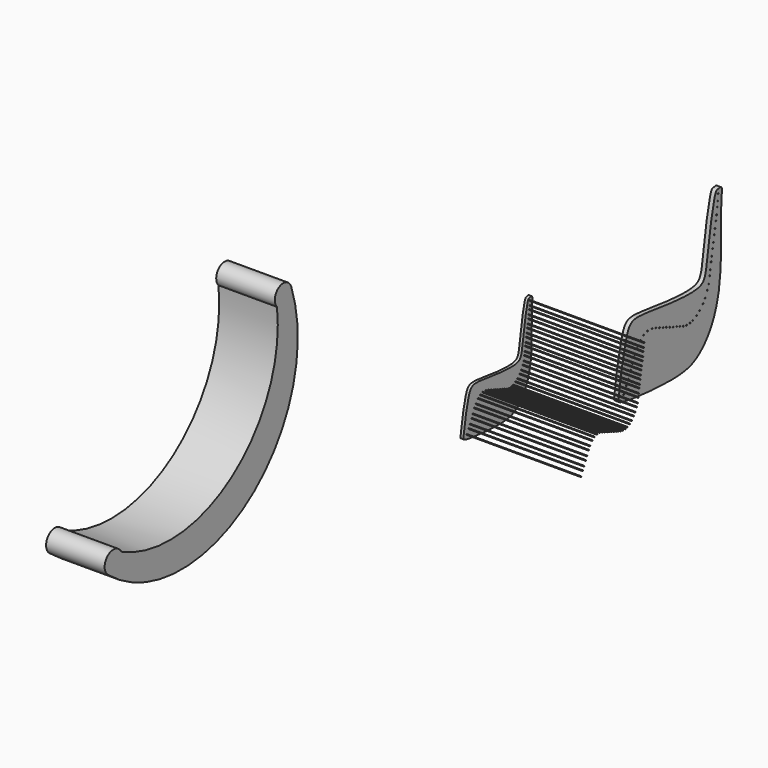
from build123d import *

# Parameters (mm, degrees)
F2_DEPTH = 127
F4_DEPTH = 12.7
F5_SCALE = 1.5
F6_DEPTH = 508


# Not quite as in the source:
# - a feature names something its author has since deleted; it is built from what else it names


with BuildPart() as f2:
    # F1 (on Right) → F2 (new body, symmetric)
    with BuildSketch(Plane.YZ):
        with BuildLine():
            ThreePointArc((-405.3666641437, -282.9348817468), (-431.1960064464, -325.2227693858), (-480.6119799614, -321.5509951115))
            ThreePointArc((-480.6119799614, -321.5509951115), (278.9839250065, -347.7055505892), (511.339366436, 375.9524822235))
            ThreePointArc((511.339366436, 375.9524822235), (513.173736402, 368.6540148527), (513.7907227287, 361.1538903865))
            ThreePointArc((513.7907227287, 361.1538903865), (484.5631181842, 318.392706642), (434.1071248055, 330.0958871841))
            ThreePointArc((434.1071248055, 330.0958871841), (189.1196757774, -218.9533749106), (-410.6203019619, -261.2133026123))
            ThreePointArc((-410.6203019619, -261.2133026123), (-406.6987393278, -271.7609420832), (-405.3666641437, -282.9348817468))
        make_face()
        with BuildLine():
            ThreePointArc((-410.6203019619, -261.2133026123), (-483.9335544164, -246.9339780219), (-480.6119799614, -321.5509951115))
            ThreePointArc((-480.6119799614, -321.5509951115), (-431.1960064464, -325.2227693858), (-405.3666641437, -282.9348817468))
            ThreePointArc((-405.3666641437, -282.9348817468), (-406.6987393278, -271.7609420832), (-410.6203019619, -261.2133026123))
        make_face()
        with BuildLine():
            ThreePointArc((513.7907227287, 361.1538903865), (513.173736402, 368.6540148527), (511.339366436, 375.9524822235))
            ThreePointArc((511.339366436, 375.9524822235), (444.4653431931, 400.6164916858), (434.1071248055, 330.0958871841))
            ThreePointArc((434.1071248055, 330.0958871841), (484.5631181842, 318.392706642), (513.7907227287, 361.1538903865))
        make_face()
    extrude(amount=F2_DEPTH, both=True)


with BuildPart() as f4:
    # F3 (on Right) → F4 (new body)
    with BuildSketch(Plane.YZ):
        with BuildLine():
            add(Edge.make_bspline(
                [(1588.1042480469, -672.3895072937), (1590.7751967656, -646.3995932049), (1611.7959010002, -517.5506212092), (1641.7401584726, -489.021724859), (1720.9312550677, -500.8093748422), (1881.0798668429, -519.9918232799), (1904.7947275082, -486.1107940737), (1911.014539794, -415.1749746357), (1934.8258228227, -286.8214563677), (1945.6474567466, -286.2346451362), (1965.0613414177, -281.763240351), (1954.2066132557, -330.1428987209), (1965.6410866407, -524.5072510181), (1926.7903882604, -626.0098057417), (1895.9895754535, -664.9340201656), (1851.033974807, -703.2355431509), (1742.9778221098, -706.2354101889), (1588.1977710336, -690.3922627167), (1587.3192204388, -680.0282912013), (1588.1042480469, -672.3895072937)],
                knots=[0, 0, 0, 0, 0.086766165, 0.1291659204, 0.191487798, 0.2795961904, 0.3179244262, 0.3798889709, 0.4579456316, 0.4772361122, 0.5017320687, 0.543105293, 0.6429735253, 0.7164751466, 0.7638864843, 0.8141635884, 0.8901962157, 0.9744982618, 1, 1, 1, 1], degree=3))
        make_face()
        with BuildLine():
            ThreePointArc((1607.8116078098, -670.6807075021), (1604.8770943632, -671.5207735855), (1606.9225230544, -669.2550945124))
            ThreePointArc((1606.9225230544, -669.2550945124), (1607.5711212565, -669.8406414186), (1607.8116078098, -670.6807075021))
        make_face(mode=Mode.SUBTRACT)
        with BuildLine():
            ThreePointArc((1617.2146263828, -651.7951774392), (1616.4601126896, -653.1465804371), (1614.9137885085, -653.2133824057))
            ThreePointArc((1614.9137885085, -653.2133824057), (1614.2090096098, -651.0816642522), (1616.3408148715, -650.3771488812))
            ThreePointArc((1616.3408148715, -650.3771488812), (1616.9786323439, -650.9623581988), (1617.2146263828, -651.7951774392))
        make_face(mode=Mode.SUBTRACT)
        with BuildLine():
            ThreePointArc((1624.441297583, -637.4331976519), (1623.6873478332, -638.7842528803), (1622.1416437494, -638.8519975557))
            ThreePointArc((1622.1416437494, -638.8519975557), (1621.4348029778, -636.7214318474), (1623.5651753051, -636.0140084515))
            ThreePointArc((1623.5651753051, -636.0140084515), (1624.2046248081, -636.5992779566), (1624.441297583, -637.4331976519))
        make_face(mode=Mode.SUBTRACT)
        with BuildLine():
            ThreePointArc((1633.4229065248, -619.2392863847), (1632.6790615082, -620.5840549591), (1631.1446041388, -620.6686038139))
            ThreePointArc((1631.1446041388, -620.6686038139), (1630.4054246212, -618.5498605326), (1632.5234552037, -617.8086413325))
            ThreePointArc((1632.5234552037, -617.8086413325), (1633.1793621654, -618.3943369861), (1633.4229065248, -619.2392863847))
        make_face(mode=Mode.SUBTRACT)
        with BuildLine():
            ThreePointArc((1640.1858726451, -604.7830555746), (1639.4584529937, -606.1173786404), (1637.9428262905, -606.2288824062))
            ThreePointArc((1637.9428262905, -606.2288824062), (1637.1518979459, -604.1289399927), (1639.251056814, -603.3359344236))
            ThreePointArc((1639.251056814, -603.3359344236), (1639.9318441237, -603.9216555131), (1640.1858726451, -604.7830555746))
        make_face(mode=Mode.SUBTRACT)
        with BuildLine():
            ThreePointArc((1648.8267409237, -585.9965814537), (1648.0802623737, -587.3429986144), (1646.5428490552, -587.4231839266))
            ThreePointArc((1646.5428490552, -587.4231839266), (1645.8151480681, -585.295071804), (1647.9458593109, -584.5750165748))
            ThreePointArc((1647.9458593109, -584.5750165748), (1648.5886691248, -585.1603997868), (1648.8267409237, -585.9965814537))
        make_face(mode=Mode.SUBTRACT)
        with BuildLine():
            ThreePointArc((1656.0821342109, -572.7840732335), (1655.2700718309, -574.1692998386), (1653.6646819307, -574.1373416705))
            ThreePointArc((1653.6646819307, -574.1373416705), (1653.147010351, -571.944986717), (1655.3428165759, -571.4421556035))
            ThreePointArc((1655.3428165759, -571.4421556035), (1655.8850740252, -572.0180227308), (1656.0821342109, -572.7840732335))
        make_face(mode=Mode.SUBTRACT)
        with BuildLine():
            ThreePointArc((1668.1439102008, -557.277738545), (1667.1696433417, -558.7420135755), (1665.4426801347, -558.4090040266))
            ThreePointArc((1665.4426801347, -558.4090040266), (1665.4394903681, -556.1496222667), (1667.6987279241, -556.1753472946))
            ThreePointArc((1667.6987279241, -556.1753472946), (1668.028413196, -556.6832947443), (1668.1439102008, -557.277738545))
        make_face(mode=Mode.SUBTRACT)
        with BuildLine():
            ThreePointArc((1680.1075762918, -548.3992204924), (1678.9093390409, -549.9382561522), (1677.1234745442, -549.1539786049))
            ThreePointArc((1677.1234745442, -549.1539786049), (1677.7903828704, -546.9893610097), (1679.9427437215, -547.6948245564))
            ThreePointArc((1679.9427437215, -547.6948245564), (1680.0658189603, -548.0375081029), (1680.1075762918, -548.3992204924))
        make_face(mode=Mode.SUBTRACT)
        with BuildLine():
            ThreePointArc((1694.1690954304, -543.8397874236), (1692.7157248498, -545.4216109121), (1691.0167608806, -544.1070870345))
            ThreePointArc((1691.0167608806, -544.1070870345), (1692.3410507485, -542.2706174181), (1694.1546434805, -543.6260677893))
            ThreePointArc((1694.1546434805, -543.6260677893), (1694.1654783221, -543.732683571), (1694.1690954304, -543.8397874236))
        make_face(mode=Mode.SUBTRACT)
        with BuildLine():
            ThreePointArc((1710.5441406901, -544.5462468817), (1708.6919971387, -545.7888023035), (1707.4253199722, -543.9530712046))
            ThreePointArc((1707.4253199722, -543.9530712046), (1709.127233525, -542.647822494), (1710.5761103558, -544.2292585082))
            ThreePointArc((1710.5761103558, -544.2292585082), (1710.5680977181, -544.3885567257), (1710.5441406901, -544.5462468817))
        make_face(mode=Mode.SUBTRACT)
        with BuildLine():
            ThreePointArc((1737.2629255193, -553.4428964877), (1735.2296018425, -554.3961653446), (1734.277468412, -552.3623097405))
            ThreePointArc((1734.277468412, -552.3623097405), (1736.0446029311, -551.3398854822), (1737.3573953003, -552.9034365583))
            ThreePointArc((1737.3573953003, -552.9034365583), (1737.3335995119, -553.1772711594), (1737.2629255193, -553.4428964877))
        make_face(mode=Mode.SUBTRACT)
        with BuildLine():
            ThreePointArc((1724.2944062995, -548.7008975511), (1722.2714523473, -549.6646490244), (1721.3000207205, -547.645371879))
            ThreePointArc((1721.3000207205, -547.645371879), (1723.0639632017, -546.6021765173), (1724.3867189937, -548.1674454253))
            ThreePointArc((1724.3867189937, -548.1674454253), (1724.3634705876, -548.438135656), (1724.2944062995, -548.7008975511))
        make_face(mode=Mode.SUBTRACT)
        with BuildLine():
            ThreePointArc((1774.5199183751, -567.3192876221), (1772.4736103417, -568.2463379373), (1771.5491941784, -566.1988385816))
            ThreePointArc((1771.5491941784, -566.1988385816), (1773.3195698429, -565.1994010322), (1774.6213353258, -566.760974609))
            ThreePointArc((1774.6213353258, -566.760974609), (1774.59577532, -567.0446993077), (1774.5199183751, -567.3192876221))
        make_face(mode=Mode.SUBTRACT)
        with BuildLine():
            ThreePointArc((1810.7484525345, -580.2102675809), (1808.6922734317, -581.1106920696), (1807.7911653811, -579.0548124418))
            ThreePointArc((1807.7911653811, -579.0548124418), (1809.5636884966, -578.0719510027), (1810.8575010331, -579.6320484112))
            ThreePointArc((1810.8575010331, -579.6320484112), (1810.830000714, -579.9262545393), (1810.7484525345, -580.2102675809))
        make_face(mode=Mode.SUBTRACT)
        with BuildLine():
            ThreePointArc((1799.5859865469, -576.0176416187), (1797.5673258198, -576.9949554391), (1796.5859372452, -574.9782725439))
            ThreePointArc((1796.5859372452, -574.9782725439), (1798.3489283907, -573.9291832582), (1799.674511417, -575.4949277293))
            ThreePointArc((1799.674511417, -575.4949277293), (1799.6522237459, -575.7600062379), (1799.5859865469, -576.0176416187))
        make_face(mode=Mode.SUBTRACT)
        with BuildLine():
            ThreePointArc((1786.6946986099, -571.6457977617), (1784.6789485496, -572.6379813997), (1783.6897110936, -570.6207838555))
            ThreePointArc((1783.6897110936, -570.6207838555), (1785.452354624, -569.5695715498), (1786.7789560498, -571.1354860379))
            ThreePointArc((1786.7789560498, -571.1354860379), (1786.7577500538, -571.3940964455), (1786.6946986099, -571.6457977617))
        make_face(mode=Mode.SUBTRACT)
        with BuildLine():
            ThreePointArc((1750.305503235, -558.148216571), (1748.2717699033, -559.0972444943), (1747.3212947938, -557.0641871096))
            ThreePointArc((1747.3212947938, -557.0641871096), (1749.0884012408, -556.0415728059), (1750.4012847713, -557.6051398958))
            ThreePointArc((1750.4012847713, -557.6051398958), (1750.3771560182, -557.8808691008), (1750.305503235, -558.148216571))
        make_face(mode=Mode.SUBTRACT)
        with BuildLine():
            ThreePointArc((1762.0275438924, -562.5443596374), (1759.9780969049, -563.4589322465), (1759.0620458975, -561.4101456388))
            ThreePointArc((1759.0620458975, -561.4101456388), (1760.8329910217, -560.4149862356), (1762.1327040518, -561.9761828632))
            ThreePointArc((1762.1327040518, -561.9761828632), (1762.1061926403, -562.2650961312), (1762.0275438924, -562.5443596374))
        make_face(mode=Mode.SUBTRACT)
        with BuildLine():
            ThreePointArc((1823.4422161957, -584.6207885167), (1821.4649270344, -585.7085956437), (1820.3978471084, -583.7200441094))
            ThreePointArc((1820.3978471084, -583.7200441094), (1822.1510800028, -582.6164313554), (1823.5028238431, -584.186327939))
            ThreePointArc((1823.5028238431, -584.186327939), (1823.487598924, -584.4056617488), (1823.4422161957, -584.6207885167))
        make_face(mode=Mode.SUBTRACT)
        with BuildLine():
            ThreePointArc((1834.6505710653, -586.4496602403), (1832.9406289999, -587.9321220896), (1831.4859352777, -586.1984954931))
            ThreePointArc((1831.4859352777, -586.1984954931), (1833.1418650629, -584.7639013207), (1834.6537277064, -586.3495984041))
            ThreePointArc((1834.6537277064, -586.3495984041), (1834.6529383499, -586.3996542116), (1834.6505710653, -586.4496602403))
        make_face(mode=Mode.SUBTRACT)
        with BuildLine():
            ThreePointArc((1847.7464040441, -585.7525070104), (1846.2773557163, -587.3355816932), (1844.5890806408, -585.9887499627))
            ThreePointArc((1844.5890806408, -585.9887499627), (1845.9014887363, -584.186016152), (1847.7217768173, -585.4739662689))
            ThreePointArc((1847.7217768173, -585.4739662689), (1847.7402352519, -585.6126933442), (1847.7464040441, -585.7525070104))
        make_face(mode=Mode.SUBTRACT)
        with BuildLine():
            ThreePointArc((1857.7834266663, -583.1956975162), (1856.4504171958, -584.7626661886), (1854.6900209083, -583.6980958622))
            ThreePointArc((1854.6900209083, -583.6980958622), (1855.6738506143, -581.6965001156), (1857.6881585927, -582.6540332958))
            ThreePointArc((1857.6881585927, -582.6540332958), (1857.7594282546, -582.9207083648), (1857.7834266663, -583.1956975162))
        make_face(mode=Mode.SUBTRACT)
        with BuildLine():
            ThreePointArc((1871.5928569434, -576.4107363499), (1870.4434710585, -577.9365844), (1868.6596761281, -577.2529354909))
            ThreePointArc((1868.6596761281, -577.2529354909), (1869.1489309279, -575.0740648383), (1871.3328687471, -575.5401798261))
            ThreePointArc((1871.3328687471, -575.5401798261), (1871.5264718698, -575.9564615092), (1871.5928569434, -576.4107363499))
        make_face(mode=Mode.SUBTRACT)
        with BuildLine():
            ThreePointArc((1882.1917912244, -568.3516339949), (1881.1589575117, -569.8390819972), (1879.4043876846, -569.3910510166))
            ThreePointArc((1879.4043876846, -569.3910510166), (1879.5556247362, -567.1598056321), (1881.7879731125, -567.2937807736))
            ThreePointArc((1881.7879731125, -567.2937807736), (1882.0874047142, -567.7854797523), (1882.1917912244, -568.3516339949))
        make_face(mode=Mode.SUBTRACT)
        with BuildLine():
            ThreePointArc((1894.2156929016, -555.8068156242), (1893.3266466588, -557.2324097457), (1891.655291517, -557.0612553979))
            ThreePointArc((1891.655291517, -557.0612553979), (1891.4012728026, -554.7994312286), (1893.6692822678, -554.6083627959))
            ThreePointArc((1893.6692822678, -554.6083627959), (1894.0726453271, -555.1482463867), (1894.2156929016, -555.8068156242))
        make_face(mode=Mode.SUBTRACT)
        with BuildLine():
            ThreePointArc((1902.3290771484, -544.2246794701), (1901.6014987395, -545.5591048547), (1900.0856867771, -545.6703502731))
            ThreePointArc((1900.0856867771, -545.6703502731), (1899.3940907259, -543.385372261), (1901.7498866849, -542.9985195585))
            ThreePointArc((1901.7498866849, -542.9985195585), (1902.1769947948, -543.5466437553), (1902.3290771484, -544.2246794701))
        make_face(mode=Mode.SUBTRACT)
        with BuildLine():
            ThreePointArc((1910.1663726807, -528.0185937881), (1909.7127981015, -529.1296155656), (1908.6112616383, -529.605763346))
            ThreePointArc((1908.6112616383, -529.605763346), (1907.1112759866, -527.4133531802), (1909.7206669429, -526.9156603755))
            ThreePointArc((1909.7206669429, -526.9156603755), (1910.0507345358, -527.4238006061), (1910.1663726807, -528.0185937881))
        make_face(mode=Mode.SUBTRACT)
        with BuildLine():
            ThreePointArc((1915.2141708374, -514.0707492828), (1914.694888062, -515.2450866326), (1913.4767620675, -515.6511554366))
            ThreePointArc((1913.4767620675, -515.6511554366), (1912.0887035421, -513.6772866434), (1914.2541449789, -512.612520065))
            ThreePointArc((1914.2541449789, -512.612520065), (1914.9526179422, -513.1978114126), (1915.2141708374, -514.0707492828))
        make_face(mode=Mode.SUBTRACT)
        with BuildLine():
            ThreePointArc((1918.8008207321, -494.809448719), (1918.3431323994, -495.9246535641), (1917.2339774609, -496.3968143195))
            ThreePointArc((1917.2339774609, -496.3968143195), (1915.6412587006, -494.5885930668), (1917.6705566059, -493.2892212342))
            ThreePointArc((1917.6705566059, -493.2892212342), (1918.4872944759, -493.8622701983), (1918.8008207321, -494.809448719))
        make_face(mode=Mode.SUBTRACT)
        with BuildLine():
            ThreePointArc((1921.0590023041, -480.197429657), (1920.5067501223, -481.4009321309), (1919.2342234633, -481.7670968197))
            ThreePointArc((1919.2342234633, -481.7670968197), (1917.9000832737, -479.9720444732), (1919.6849809054, -478.6243488781))
            ThreePointArc((1919.6849809054, -478.6243488781), (1920.6671304924, -479.1530975809), (1921.0590023041, -480.197429657))
        make_face(mode=Mode.SUBTRACT)
        with BuildLine():
            ThreePointArc((1923.7158197403, -461.0689580441), (1923.2804559667, -462.1610836622), (1922.2131572323, -462.6541895256))
            ThreePointArc((1922.2131572323, -462.6541895256), (1920.5641059915, -460.7980492071), (1922.7413231088, -459.6045868069))
            ThreePointArc((1922.7413231088, -459.6045868069), (1923.4499284376, -460.1894657466), (1923.7158197403, -461.0689580441))
        make_face(mode=Mode.SUBTRACT)
        with BuildLine():
            ThreePointArc((1926.3485569, -447.9891061783), (1925.8205188656, -449.1713483673), (1924.5876793018, -449.5671101258))
            ThreePointArc((1924.5876793018, -449.5671101258), (1923.2029043191, -447.6852694053), (1925.1932534089, -446.4615714233))
            ThreePointArc((1925.1932534089, -446.4615714233), (1926.0272062214, -447.0314934455), (1926.3485569, -447.9891061783))
        make_face(mode=Mode.SUBTRACT)
        with BuildLine():
            ThreePointArc((1929.5365709305, -429.7904670238), (1929.1664541348, -430.8093558224), (1928.2286850927, -431.3531481078))
            ThreePointArc((1928.2286850927, -431.3531481078), (1926.3912865875, -429.4847478867), (1928.7985579623, -428.4493749194))
            ThreePointArc((1928.7985579623, -428.4493749194), (1929.3398830877, -429.0250927406), (1929.5365709305, -429.7904670238))
        make_face(mode=Mode.SUBTRACT)
        with BuildLine():
            ThreePointArc((1932.1932691574, -415.0456190109), (1931.8391675323, -416.0450612048), (1930.9348317416, -416.5986399592))
            ThreePointArc((1930.9348317416, -416.5986399592), (1929.0381181676, -414.7953658908), (1931.4019907701, -413.672233634))
            ThreePointArc((1931.4019907701, -413.672233634), (1931.981297794, -414.2531057808), (1932.1932691574, -415.0456190109))
        make_face(mode=Mode.SUBTRACT)
        with BuildLine():
            ThreePointArc((1935.2486032486, -396.8470096588), (1934.7744827296, -397.9786201843), (1933.6353215084, -398.4343002913))
            ThreePointArc((1933.6353215084, -398.4343002913), (1932.090167208, -396.6182822966), (1934.0890138648, -395.3182687538))
            ThreePointArc((1934.0890138648, -395.3182687538), (1934.9259084417, -395.8876223161), (1935.2486032486, -396.8470096588))
        make_face(mode=Mode.SUBTRACT)
        with BuildLine():
            ThreePointArc((1937.9053014755, -381.9693028927), (1937.304897939, -383.2126036696), (1935.9578409126, -383.5154544516))
            ThreePointArc((1935.9578409126, -383.5154544516), (1934.7545910915, -381.6926631534), (1936.5103263786, -380.3935204167))
            ThreePointArc((1936.5103263786, -380.3935204167), (1937.506453976, -380.9170379626), (1937.9053014755, -381.9693028927))
        make_face(mode=Mode.SUBTRACT)
        with BuildLine():
            ThreePointArc((1940.9605163574, -364.0363514423), (1940.4704353537, -365.1834468161), (1939.3027805507, -365.6222969589))
            ThreePointArc((1939.3027805507, -365.6222969589), (1937.813259898, -363.7408585704), (1939.8877364315, -362.5346126184))
            ThreePointArc((1939.8877364315, -362.5346126184), (1940.6647737587, -363.1135735351), (1940.9605163574, -364.0363514423))
        make_face(mode=Mode.SUBTRACT)
        with BuildLine():
            ThreePointArc((1943.54914608, -349.4700193405), (1943.0669204791, -350.6095476432), (1941.9132093837, -351.0567802351))
            ThreePointArc((1941.9132093837, -351.0567802351), (1940.3932351212, -349.2245742055), (1942.4002868176, -347.9443225969))
            ThreePointArc((1942.4002868176, -347.9443225969), (1943.2298137387, -348.5150811019), (1943.54914608, -349.4700193405))
        make_face(mode=Mode.SUBTRACT)
        with BuildLine():
            ThreePointArc((1945.9186691284, -330.8295309544), (1945.5021356618, -331.9014421576), (1944.4711181015, -332.4108501931))
            ThreePointArc((1944.4711181015, -332.4108501931), (1942.7542181681, -330.6468237606), (1944.8289835188, -329.3221036484))
            ThreePointArc((1944.8289835188, -329.3221036484), (1945.6177220023, -329.89951055), (1945.9186691284, -330.8295309544))
        make_face(mode=Mode.SUBTRACT)
        with BuildLine():
            ThreePointArc((1947.6563829422, -316.1382973194), (1947.1969140718, -317.2553031478), (1946.0844748846, -317.7257207479))
            ThreePointArc((1946.0844748846, -317.7257207479), (1944.4899028912, -315.9740467533), (1946.4108634021, -314.5880697184))
            ThreePointArc((1946.4108634021, -314.5880697184), (1947.3064309675, -315.1439980008), (1947.6563829422, -316.1382973194))
        make_face(mode=Mode.SUBTRACT)
        with BuildLine():
            ThreePointArc((1949.394096756, -297.6557910442), (1948.9837865127, -298.7208640589), (1947.964955935, -299.2353728308))
            ThreePointArc((1947.964955935, -299.2353728308), (1946.2268670936, -297.498913883), (1948.2725243289, -296.1382048863))
            ThreePointArc((1948.2725243289, -296.1382048863), (1949.0832753122, -296.71226144), (1949.394096756, -297.6557910442))
        make_face(mode=Mode.SUBTRACT)
    extrude(amount=F4_DEPTH)


with BuildPart() as f5_1:
    # F5: copy of F4
    add(f4.part.scale(F5_SCALE).moved(Location((0, 39.0431753289, 147.3139180805))))


with BuildPart() as f6:
    # F3 (on Right) → F6 (new body)
    with BuildSketch(Plane.YZ):
        with BuildLine():
            add(Edge.make_bspline(
                [(1820.3978471084, -583.7200441094), (1821.4075825794, -584.0409260769), (1822.4220123868, -584.3429556702), (1823.4422161957, -584.6207885167)],
                knots=[0.4538628517, 0.4538628517, 0.4538628517, 0.4538628517, 0.4591945229, 0.4591945229, 0.4591945229, 0.4591945229], degree=3))
            ThreePointArc((1820.3978471084, -583.7200441094), (1821.4649270344, -585.7085956437), (1823.4422161957, -584.6207885167))
        make_face()
        with BuildLine():
            ThreePointArc((1823.5028238431, -584.186327939), (1822.1510800028, -582.6164313554), (1820.3978471084, -583.7200441094))
            add(Edge.make_bspline(
                [(1820.3978471084, -583.7200441094), (1821.4075825794, -584.0409260769), (1822.4220123868, -584.3429556702), (1823.4422161957, -584.6207885167)],
                knots=[0.4538628517, 0.4538628517, 0.4538628517, 0.4538628517, 0.4591945229, 0.4591945229, 0.4591945229, 0.4591945229], degree=3))
            ThreePointArc((1823.4422161957, -584.6207885167), (1823.487598924, -584.4056617488), (1823.5028238431, -584.186327939))
        make_face()
    extrude(amount=F6_DEPTH)


with BuildPart() as f6b:
    # F3 (on Right) → F6, piece 2 (new body)
    with BuildSketch(Plane.YZ):
        with BuildLine():
            add(Edge.make_bspline(
                [(1721.3000207205, -547.645371879), (1722.301254183, -547.9890576359), (1723.2993342363, -548.3423273885), (1724.2944062995, -548.7008975511)],
                knots=[0.2789234558, 0.2789234558, 0.2789234558, 0.2789234558, 0.2839665966, 0.2839665966, 0.2839665966, 0.2839665966], degree=3))
            ThreePointArc((1721.3000207205, -547.645371879), (1722.2714523473, -549.6646490244), (1724.2944062995, -548.7008975511))
        make_face()
        with BuildLine():
            ThreePointArc((1724.3867189937, -548.1674454253), (1723.0639632017, -546.6021765173), (1721.3000207205, -547.645371879))
            add(Edge.make_bspline(
                [(1721.3000207205, -547.645371879), (1722.301254183, -547.9890576359), (1723.2993342363, -548.3423273885), (1724.2944062995, -548.7008975511)],
                knots=[0.2789234558, 0.2789234558, 0.2789234558, 0.2789234558, 0.2839665966, 0.2839665966, 0.2839665966, 0.2839665966], degree=3))
            ThreePointArc((1724.2944062995, -548.7008975511), (1724.3634705876, -548.438135656), (1724.3867189937, -548.1674454253))
        make_face()
    extrude(amount=F6_DEPTH)


with BuildPart() as f6c:
    # F3 (on Right) → F6, piece 3 (new body)
    with BuildSketch(Plane.YZ):
        with BuildLine():
            ThreePointArc((1871.3328687471, -575.5401798261), (1869.1489309279, -575.0740648383), (1868.6596761281, -577.2529354909))
            add(Edge.make_bspline(
                [(1868.6596761281, -577.2529354909), (1869.5596900164, -576.7031584925), (1870.4505050114, -576.1319804525), (1871.3328687471, -575.5401798261)],
                knots=[0.5375577553, 0.5375577553, 0.5375577553, 0.5375577553, 0.5428134997, 0.5428134997, 0.5428134997, 0.5428134997], degree=3))
        make_face()
        with BuildLine():
            add(Edge.make_bspline(
                [(1868.6596761281, -577.2529354909), (1869.5596900164, -576.7031584925), (1870.4505050114, -576.1319804525), (1871.3328687471, -575.5401798261)],
                knots=[0.5375577553, 0.5375577553, 0.5375577553, 0.5375577553, 0.5428134997, 0.5428134997, 0.5428134997, 0.5428134997], degree=3))
            ThreePointArc((1868.6596761281, -577.2529354909), (1870.4434710585, -577.9365844), (1871.5928569434, -576.4107363499))
            ThreePointArc((1871.5928569434, -576.4107363499), (1871.5264718698, -575.9564615092), (1871.3328687471, -575.5401798261))
        make_face()
    extrude(amount=F6_DEPTH)


with BuildPart() as f6d:
    # F3 (on Right) → F6, piece 4 (new body)
    with BuildSketch(Plane.YZ):
        with BuildLine():
            add(Edge.make_bspline(
                [(1783.6897110936, -570.6207838555), (1784.6914397652, -570.966046895), (1785.6931392628, -571.3071272185), (1786.6946986099, -571.6457977617)],
                knots=[0.3882589147, 0.3882589147, 0.3882589147, 0.3882589147, 0.3936211809, 0.3936211809, 0.3936211809, 0.3936211809], degree=3))
            ThreePointArc((1783.6897110936, -570.6207838555), (1784.6789485496, -572.6379813997), (1786.6946986099, -571.6457977617))
        make_face()
        with BuildLine():
            ThreePointArc((1786.7789560498, -571.1354860379), (1785.452354624, -569.5695715498), (1783.6897110936, -570.6207838555))
            add(Edge.make_bspline(
                [(1783.6897110936, -570.6207838555), (1784.6914397652, -570.966046895), (1785.6931392628, -571.3071272185), (1786.6946986099, -571.6457977617)],
                knots=[0.3882589147, 0.3882589147, 0.3882589147, 0.3882589147, 0.3936211809, 0.3936211809, 0.3936211809, 0.3936211809], degree=3))
            ThreePointArc((1786.6946986099, -571.6457977617), (1786.7577500538, -571.3940964455), (1786.7789560498, -571.1354860379))
        make_face()
    extrude(amount=F6_DEPTH)


with BuildPart() as f6e:
    # F3 (on Right) → F6, piece 5 (new body)
    with BuildSketch(Plane.YZ):
        with BuildLine():
            ThreePointArc((1679.9427437215, -547.6948245564), (1677.7903828704, -546.9893610097), (1677.1234745442, -549.1539786049))
            add(Edge.make_bspline(
                [(1677.1234745442, -549.1539786049), (1678.0482740292, -548.6325524406), (1678.9888013985, -548.1461973372), (1679.9427437215, -547.6948245564)],
                knots=[0.2062695622, 0.2062695622, 0.2062695622, 0.2062695622, 0.2112171929, 0.2112171929, 0.2112171929, 0.2112171929], degree=3))
        make_face()
        with BuildLine():
            add(Edge.make_bspline(
                [(1677.1234745442, -549.1539786049), (1678.0482740292, -548.6325524406), (1678.9888013985, -548.1461973372), (1679.9427437215, -547.6948245564)],
                knots=[0.2062695622, 0.2062695622, 0.2062695622, 0.2062695622, 0.2112171929, 0.2112171929, 0.2112171929, 0.2112171929], degree=3))
            ThreePointArc((1677.1234745442, -549.1539786049), (1678.9093390409, -549.9382561522), (1680.1075762918, -548.3992204924))
            ThreePointArc((1680.1075762918, -548.3992204924), (1680.0658189603, -548.0375081029), (1679.9427437215, -547.6948245564))
        make_face()
    extrude(amount=F6_DEPTH)


with BuildPart() as f6f:
    # F3 (on Right) → F6, piece 6 (new body)
    with BuildSketch(Plane.YZ):
        with BuildLine():
            add(Edge.make_bspline(
                [(1747.3212947938, -557.0641871096), (1748.3176839229, -557.4246394513), (1749.3123484781, -557.7857334801), (1750.305503235, -558.148216571)],
                knots=[0.3236773066, 0.3236773066, 0.3236773066, 0.3236773066, 0.3289209623, 0.3289209623, 0.3289209623, 0.3289209623], degree=3))
            ThreePointArc((1747.3212947938, -557.0641871096), (1748.2717699033, -559.0972444943), (1750.305503235, -558.148216571))
        make_face()
        with BuildLine():
            ThreePointArc((1750.4012847713, -557.6051398958), (1749.0884012408, -556.0415728059), (1747.3212947938, -557.0641871096))
            add(Edge.make_bspline(
                [(1747.3212947938, -557.0641871096), (1748.3176839229, -557.4246394513), (1749.3123484781, -557.7857334801), (1750.305503235, -558.148216571)],
                knots=[0.3236773066, 0.3236773066, 0.3236773066, 0.3236773066, 0.3289209623, 0.3289209623, 0.3289209623, 0.3289209623], degree=3))
            ThreePointArc((1750.305503235, -558.148216571), (1750.3771560182, -557.8808691008), (1750.4012847713, -557.6051398958))
        make_face()
    extrude(amount=F6_DEPTH)


with BuildPart() as f6g:
    # F3 (on Right) → F6, piece 7 (new body)
    with BuildSketch(Plane.YZ):
        with BuildLine():
            ThreePointArc((1901.7498866849, -542.9985195585), (1899.3940907259, -543.385372261), (1900.0856867771, -545.6703502731))
            add(Edge.make_bspline(
                [(1900.0856867771, -545.6703502731), (1900.6528416657, -544.7888177122), (1901.2076873649, -543.8979832292), (1901.7498866849, -542.9985195585)],
                knots=[0.6075663861, 0.6075663861, 0.6075663861, 0.6075663861, 0.6122541375, 0.6122541375, 0.6122541375, 0.6122541375], degree=3))
        make_face()
        with BuildLine():
            add(Edge.make_bspline(
                [(1900.0856867771, -545.6703502731), (1900.6528416657, -544.7888177122), (1901.2076873649, -543.8979832292), (1901.7498866849, -542.9985195585)],
                knots=[0.6075663861, 0.6075663861, 0.6075663861, 0.6075663861, 0.6122541375, 0.6122541375, 0.6122541375, 0.6122541375], degree=3))
            ThreePointArc((1900.0856867771, -545.6703502731), (1901.6014987395, -545.5591048547), (1902.3290771484, -544.2246794701))
            ThreePointArc((1902.3290771484, -544.2246794701), (1902.1769947948, -543.5466437553), (1901.7498866849, -542.9985195585))
        make_face()
    extrude(amount=F6_DEPTH)


with BuildPart() as f6h:
    # F3 (on Right) → F6, piece 8 (new body)
    with BuildSketch(Plane.YZ):
        with BuildLine():
            add(Edge.make_bspline(
                [(1807.7911653811, -579.0548124418), (1808.7764327991, -579.4380655803), (1809.7618397246, -579.8249768252), (1810.7484525345, -580.2102675809)],
                knots=[0.4313756155, 0.4313756155, 0.4313756155, 0.4313756155, 0.4366853228, 0.4366853228, 0.4366853228, 0.4366853228], degree=3))
            ThreePointArc((1807.7911653811, -579.0548124418), (1808.6922734317, -581.1106920696), (1810.7484525345, -580.2102675809))
        make_face()
        with BuildLine():
            ThreePointArc((1810.8575010331, -579.6320484112), (1809.5636884966, -578.0719510027), (1807.7911653811, -579.0548124418))
            add(Edge.make_bspline(
                [(1807.7911653811, -579.0548124418), (1808.7764327991, -579.4380655803), (1809.7618397246, -579.8249768252), (1810.7484525345, -580.2102675809)],
                knots=[0.4313756155, 0.4313756155, 0.4313756155, 0.4313756155, 0.4366853228, 0.4366853228, 0.4366853228, 0.4366853228], degree=3))
            ThreePointArc((1810.7484525345, -580.2102675809), (1810.830000714, -579.9262545393), (1810.8575010331, -579.6320484112))
        make_face()
    extrude(amount=F6_DEPTH)


with BuildPart() as f6i:
    # F3 (on Right) → F6, piece 9 (new body)
    with BuildSketch(Plane.YZ):
        with BuildLine():
            ThreePointArc((1694.1546434805, -543.6260677893), (1692.3410507485, -542.2706174181), (1691.0167608806, -544.1070870345))
            add(Edge.make_bspline(
                [(1691.0167608806, -544.1070870345), (1692.0585297188, -543.9107522467), (1693.1053078651, -543.7504438542), (1694.1546434804, -543.6260677893)],
                knots=[0.2296065018, 0.2296065018, 0.2296065018, 0.2296065018, 0.2346512605, 0.2346512605, 0.2346512605, 0.2346512605], degree=3))
        make_face()
        with BuildLine():
            add(Edge.make_bspline(
                [(1691.0167608806, -544.1070870345), (1692.0585297188, -543.9107522467), (1693.1053078651, -543.7504438542), (1694.1546434804, -543.6260677893)],
                knots=[0.2296065018, 0.2296065018, 0.2296065018, 0.2296065018, 0.2346512605, 0.2346512605, 0.2346512605, 0.2346512605], degree=3))
            ThreePointArc((1691.0167608806, -544.1070870345), (1692.7157248498, -545.4216109121), (1694.1690954304, -543.8397874236))
            ThreePointArc((1694.1690954304, -543.8397874236), (1694.1654783221, -543.732683571), (1694.1546434805, -543.6260677893))
        make_face()
    extrude(amount=F6_DEPTH)


with BuildPart() as f6j:
    # F3 (on Right) → F6, piece 10 (new body)
    with BuildSketch(Plane.YZ):
        with BuildLine():
            ThreePointArc((1667.6987279241, -556.1753472946), (1665.4394903681, -556.1496222667), (1665.4426801347, -558.4090040266))
            add(Edge.make_bspline(
                [(1665.4426801347, -558.4090040266), (1666.179665914, -557.6416881512), (1666.9315889309, -556.8962765178), (1667.6987279241, -556.1753472946)],
                knots=[0.183522289, 0.183522289, 0.183522289, 0.183522289, 0.1882590347, 0.1882590347, 0.1882590347, 0.1882590347], degree=3))
        make_face()
        with BuildLine():
            add(Edge.make_bspline(
                [(1665.4426801347, -558.4090040266), (1666.179665914, -557.6416881512), (1666.9315889309, -556.8962765178), (1667.6987279241, -556.1753472946)],
                knots=[0.183522289, 0.183522289, 0.183522289, 0.183522289, 0.1882590347, 0.1882590347, 0.1882590347, 0.1882590347], degree=3))
            ThreePointArc((1665.4426801347, -558.4090040266), (1667.1696433417, -558.7420135755), (1668.1439102008, -557.277738545))
            ThreePointArc((1668.1439102008, -557.277738545), (1668.028413196, -556.6832947443), (1667.6987279241, -556.1753472946))
        make_face()
    extrude(amount=F6_DEPTH)


with BuildPart() as f6k:
    # F3 (on Right) → F6, piece 11 (new body)
    with BuildSketch(Plane.YZ):
        with BuildLine():
            ThreePointArc((1834.6537277064, -586.3495984041), (1833.1418650629, -584.7639013207), (1831.4859352777, -586.1984954931))
            add(Edge.make_bspline(
                [(1831.4859352776, -586.1984954931), (1832.5348950411, -586.316218019), (1833.59059936, -586.3995479104), (1834.6505710653, -586.4496602403)],
                knots=[0.4729735848, 0.4729735848, 0.4729735848, 0.4729735848, 0.4782675205, 0.4782675205, 0.4782675205, 0.4782675205], degree=3))
            ThreePointArc((1834.6505710653, -586.4496602403), (1834.6529383499, -586.3996542116), (1834.6537277064, -586.3495984041))
        make_face()
        with BuildLine():
            add(Edge.make_bspline(
                [(1831.4859352776, -586.1984954931), (1832.5348950411, -586.316218019), (1833.59059936, -586.3995479104), (1834.6505710653, -586.4496602403)],
                knots=[0.4729735848, 0.4729735848, 0.4729735848, 0.4729735848, 0.4782675205, 0.4782675205, 0.4782675205, 0.4782675205], degree=3))
            ThreePointArc((1831.4859352777, -586.1984954931), (1832.9406289999, -587.9321220896), (1834.6505710653, -586.4496602403))
        make_face()
    extrude(amount=F6_DEPTH)


with BuildPart() as f6l:
    # F3 (on Right) → F6, piece 12 (new body)
    with BuildSketch(Plane.YZ):
        with BuildLine():
            ThreePointArc((1647.9458593109, -584.5750165748), (1645.8151480681, -585.295071804), (1646.5428490552, -587.4231839266))
            add(Edge.make_bspline(
                [(1646.5428490552, -587.4231839266), (1647.004134617, -586.4701223305), (1647.4713034908, -585.5206199894), (1647.9458593109, -584.5750165748)],
                knots=[0.1330867666, 0.1330867666, 0.1330867666, 0.1330867666, 0.1376895871, 0.1376895871, 0.1376895871, 0.1376895871], degree=3))
        make_face()
        with BuildLine():
            add(Edge.make_bspline(
                [(1646.5428490552, -587.4231839266), (1647.004134617, -586.4701223305), (1647.4713034908, -585.5206199894), (1647.9458593109, -584.5750165748)],
                knots=[0.1330867666, 0.1330867666, 0.1330867666, 0.1330867666, 0.1376895871, 0.1376895871, 0.1376895871, 0.1376895871], degree=3))
            ThreePointArc((1646.5428490552, -587.4231839266), (1648.0802623737, -587.3429986144), (1648.8267409237, -585.9965814537))
            ThreePointArc((1648.8267409237, -585.9965814537), (1648.5886691248, -585.1603997868), (1647.9458593109, -584.5750165748))
        make_face()
    extrude(amount=F6_DEPTH)


with BuildPart() as f6m:
    # F3 (on Right) → F6, piece 13 (new body)
    with BuildSketch(Plane.YZ):
        with BuildLine():
            add(Edge.make_bspline(
                [(1771.5491941784, -566.1988385816), (1772.539760561, -566.5751741962), (1773.5299541495, -566.9490018157), (1774.5199183751, -567.3192876221)],
                knots=[0.3665992293, 0.3665992293, 0.3665992293, 0.3665992293, 0.3718970072, 0.3718970072, 0.3718970072, 0.3718970072], degree=3))
            ThreePointArc((1771.5491941784, -566.1988385816), (1772.4736103417, -568.2463379373), (1774.5199183751, -567.3192876221))
        make_face()
        with BuildLine():
            ThreePointArc((1774.6213353258, -566.760974609), (1773.3195698429, -565.1994010322), (1771.5491941784, -566.1988385816))
            add(Edge.make_bspline(
                [(1771.5491941784, -566.1988385816), (1772.539760561, -566.5751741962), (1773.5299541495, -566.9490018157), (1774.5199183751, -567.3192876221)],
                knots=[0.3665992293, 0.3665992293, 0.3665992293, 0.3665992293, 0.3718970072, 0.3718970072, 0.3718970072, 0.3718970072], degree=3))
            ThreePointArc((1774.5199183751, -567.3192876221), (1774.59577532, -567.0446993077), (1774.6213353258, -566.760974609))
        make_face()
    extrude(amount=F6_DEPTH)


with BuildPart() as f6n:
    # F3 (on Right) → F6, piece 14 (new body)
    with BuildSketch(Plane.YZ):
        with BuildLine():
            ThreePointArc((1762.1327040518, -561.9761828632), (1760.8329910217, -560.4149862356), (1759.0620458975, -561.4101456388))
            add(Edge.make_bspline(
                [(1759.0620458975, -561.4101456388), (1760.0514591782, -561.7867537842), (1761.0399116717, -562.1651627156), (1762.0275438924, -562.5443596374)],
                knots=[0.3443917131, 0.3443917131, 0.3443917131, 0.3443917131, 0.3496533354, 0.3496533354, 0.3496533354, 0.3496533354], degree=3))
            ThreePointArc((1762.0275438924, -562.5443596374), (1762.1061926403, -562.2650961312), (1762.1327040518, -561.9761828632))
        make_face()
        with BuildLine():
            add(Edge.make_bspline(
                [(1759.0620458975, -561.4101456388), (1760.0514591782, -561.7867537842), (1761.0399116717, -562.1651627156), (1762.0275438924, -562.5443596374)],
                knots=[0.3443917131, 0.3443917131, 0.3443917131, 0.3443917131, 0.3496533354, 0.3496533354, 0.3496533354, 0.3496533354], degree=3))
            ThreePointArc((1759.0620458975, -561.4101456388), (1759.9780969049, -563.4589322465), (1762.0275438924, -562.5443596374))
        make_face()
    extrude(amount=F6_DEPTH)


with BuildPart() as f6o:
    # F3 (on Right) → F6, piece 15 (new body)
    with BuildSketch(Plane.YZ):
        with BuildLine():
            add(Edge.make_bspline(
                [(1734.277468412, -552.3623097405), (1735.275114839, -552.7247706174), (1736.2701992914, -553.0847298639), (1737.2629255192, -553.4428964877)],
                knots=[0.3009958723, 0.3009958723, 0.3009958723, 0.3009958723, 0.3061482173, 0.3061482173, 0.3061482173, 0.3061482173], degree=3))
            ThreePointArc((1734.277468412, -552.3623097405), (1735.2296018425, -554.3961653446), (1737.2629255193, -553.4428964877))
        make_face()
        with BuildLine():
            ThreePointArc((1737.3573953003, -552.9034365583), (1736.0446029311, -551.3398854822), (1734.277468412, -552.3623097405))
            add(Edge.make_bspline(
                [(1734.277468412, -552.3623097405), (1735.275114839, -552.7247706174), (1736.2701992914, -553.0847298639), (1737.2629255192, -553.4428964877)],
                knots=[0.3009958723, 0.3009958723, 0.3009958723, 0.3009958723, 0.3061482173, 0.3061482173, 0.3061482173, 0.3061482173], degree=3))
            ThreePointArc((1737.2629255193, -553.4428964877), (1737.3335995119, -553.1772711594), (1737.3573953003, -552.9034365583))
        make_face()
    extrude(amount=F6_DEPTH)


with BuildPart() as f6p:
    # F3 (on Right) → F6, piece 16 (new body)
    with BuildSketch(Plane.YZ):
        with BuildLine():
            ThreePointArc((1710.5761103558, -544.2292585082), (1709.127233525, -542.647822494), (1707.4253199722, -543.9530712046))
            add(Edge.make_bspline(
                [(1707.4253199722, -543.9530712046), (1708.4687699576, -544.1226015055), (1709.5083268951, -544.3217986405), (1710.5441406901, -544.5462468817)],
                knots=[0.2559799061, 0.2559799061, 0.2559799061, 0.2559799061, 0.2610743804, 0.2610743804, 0.2610743804, 0.2610743804], degree=3))
            ThreePointArc((1710.5441406901, -544.5462468817), (1710.5680977181, -544.3885567257), (1710.5761103558, -544.2292585082))
        make_face()
        with BuildLine():
            add(Edge.make_bspline(
                [(1707.4253199722, -543.9530712046), (1708.4687699576, -544.1226015055), (1709.5083268951, -544.3217986405), (1710.5441406901, -544.5462468817)],
                knots=[0.2559799061, 0.2559799061, 0.2559799061, 0.2559799061, 0.2610743804, 0.2610743804, 0.2610743804, 0.2610743804], degree=3))
            ThreePointArc((1707.4253199722, -543.9530712046), (1708.6919971387, -545.7888023035), (1710.5441406901, -544.5462468817))
        make_face()
    extrude(amount=F6_DEPTH)


with BuildPart() as f6q:
    # F3 (on Right) → F6, piece 17 (new body)
    with BuildSketch(Plane.YZ):
        with BuildLine():
            ThreePointArc((1847.7217768173, -585.4739662689), (1845.9014887363, -584.186016152), (1844.5890806408, -585.9887499627))
            add(Edge.make_bspline(
                [(1844.5890806408, -585.9887499627), (1845.6374509964, -585.8455582895), (1846.6824761461, -585.6735875134), (1847.7217768173, -585.4739662689)],
                knots=[0.494731102, 0.494731102, 0.494731102, 0.494731102, 0.4999543604, 0.4999543604, 0.4999543604, 0.4999543604], degree=3))
        make_face()
        with BuildLine():
            add(Edge.make_bspline(
                [(1844.5890806408, -585.9887499627), (1845.6374509964, -585.8455582895), (1846.6824761461, -585.6735875134), (1847.7217768173, -585.4739662689)],
                knots=[0.494731102, 0.494731102, 0.494731102, 0.494731102, 0.4999543604, 0.4999543604, 0.4999543604, 0.4999543604], degree=3))
            ThreePointArc((1844.5890806408, -585.9887499627), (1846.2773557163, -587.3355816932), (1847.7464040441, -585.7525070104))
            ThreePointArc((1847.7464040441, -585.7525070104), (1847.7402352519, -585.6126933442), (1847.7217768173, -585.4739662689))
        make_face()
    extrude(amount=F6_DEPTH)


with BuildPart() as f6r:
    # F3 (on Right) → F6, piece 18 (new body)
    with BuildSketch(Plane.YZ):
        with BuildLine():
            add(Edge.make_bspline(
                [(1891.655291517, -557.0612553979), (1892.3364621168, -556.255622779), (1893.0080491464, -555.4378132603), (1893.6692822678, -554.6083627959)],
                knots=[0.5862673742, 0.5862673742, 0.5862673742, 0.5862673742, 0.5910697824, 0.5910697824, 0.5910697824, 0.5910697824], degree=3))
            ThreePointArc((1891.655291517, -557.0612553979), (1893.3266466588, -557.2324097457), (1894.2156929016, -555.8068156242))
            ThreePointArc((1894.2156929016, -555.8068156242), (1894.0726453271, -555.1482463867), (1893.6692822678, -554.6083627959))
        make_face()
        with BuildLine():
            ThreePointArc((1893.6692822678, -554.6083627959), (1891.4012728026, -554.7994312286), (1891.655291517, -557.0612553979))
            add(Edge.make_bspline(
                [(1891.655291517, -557.0612553979), (1892.3364621168, -556.255622779), (1893.0080491464, -555.4378132603), (1893.6692822678, -554.6083627959)],
                knots=[0.5862673742, 0.5862673742, 0.5862673742, 0.5862673742, 0.5910697824, 0.5910697824, 0.5910697824, 0.5910697824], degree=3))
        make_face()
    extrude(amount=F6_DEPTH)


with BuildPart() as f6s:
    # F3 (on Right) → F6, piece 19 (new body)
    with BuildSketch(Plane.YZ):
        with BuildLine():
            ThreePointArc((1799.674511417, -575.4949277293), (1798.3489283907, -573.9291832582), (1796.5859372452, -574.9782725439))
            add(Edge.make_bspline(
                [(1796.5859372452, -574.9782725439), (1797.5864977359, -575.3206964932), (1798.5865512875, -575.6665598672), (1799.5859865469, -576.0176416187)],
                knots=[0.411288702, 0.411288702, 0.411288702, 0.411288702, 0.4166570277, 0.4166570277, 0.4166570277, 0.4166570277], degree=3))
            ThreePointArc((1799.5859865469, -576.0176416187), (1799.6522237459, -575.7600062379), (1799.674511417, -575.4949277293))
        make_face()
        with BuildLine():
            add(Edge.make_bspline(
                [(1796.5859372452, -574.9782725439), (1797.5864977359, -575.3206964932), (1798.5865512875, -575.6665598672), (1799.5859865469, -576.0176416187)],
                knots=[0.411288702, 0.411288702, 0.411288702, 0.411288702, 0.4166570277, 0.4166570277, 0.4166570277, 0.4166570277], degree=3))
            ThreePointArc((1796.5859372452, -574.9782725439), (1797.5673258198, -576.9949554391), (1799.5859865469, -576.0176416187))
        make_face()
    extrude(amount=F6_DEPTH)


with BuildPart() as f6t:
    # F3 (on Right) → F6, piece 20 (new body)
    with BuildSketch(Plane.YZ):
        with BuildLine():
            ThreePointArc((1881.7879731125, -567.2937807736), (1879.5556247362, -567.1598056321), (1879.4043876846, -569.3910510166))
            add(Edge.make_bspline(
                [(1879.4043876846, -569.3910510166), (1880.2049742944, -568.7084096697), (1880.999797613, -568.0091144551), (1881.7879731125, -567.2937807736)],
                knots=[0.5592882421, 0.5592882421, 0.5592882421, 0.5592882421, 0.5643170978, 0.5643170978, 0.5643170978, 0.5643170978], degree=3))
        make_face()
        with BuildLine():
            add(Edge.make_bspline(
                [(1879.4043876846, -569.3910510166), (1880.2049742944, -568.7084096697), (1880.999797613, -568.0091144551), (1881.7879731125, -567.2937807736)],
                knots=[0.5592882421, 0.5592882421, 0.5592882421, 0.5592882421, 0.5643170978, 0.5643170978, 0.5643170978, 0.5643170978], degree=3))
            ThreePointArc((1879.4043876846, -569.3910510166), (1881.1589575117, -569.8390819972), (1882.1917912244, -568.3516339949))
            ThreePointArc((1882.1917912244, -568.3516339949), (1882.0874047142, -567.7854797523), (1881.7879731125, -567.2937807736))
        make_face()
    extrude(amount=F6_DEPTH)


with BuildPart() as f6u:
    # F3 (on Right) → F6, piece 21 (new body)
    with BuildSketch(Plane.YZ):
        with BuildLine():
            ThreePointArc((1655.3428165759, -571.4421556035), (1653.147010351, -571.944986717), (1653.6646819307, -574.1373416705))
            add(Edge.make_bspline(
                [(1653.6646819307, -574.1373416705), (1654.2116326844, -573.232272674), (1654.7709273909, -572.3331049131), (1655.3428165759, -571.4421556035)],
                knots=[0.1549201485, 0.1549201485, 0.1549201485, 0.1549201485, 0.1594913653, 0.1594913653, 0.1594913653, 0.1594913653], degree=3))
        make_face()
        with BuildLine():
            add(Edge.make_bspline(
                [(1653.6646819307, -574.1373416705), (1654.2116326844, -573.232272674), (1654.7709273909, -572.3331049131), (1655.3428165759, -571.4421556035)],
                knots=[0.1549201485, 0.1549201485, 0.1549201485, 0.1549201485, 0.1594913653, 0.1594913653, 0.1594913653, 0.1594913653], degree=3))
            ThreePointArc((1653.6646819307, -574.1373416705), (1655.2700718309, -574.1692998386), (1656.0821342109, -572.7840732335))
            ThreePointArc((1656.0821342109, -572.7840732335), (1655.8850740252, -572.0180227308), (1655.3428165759, -571.4421556035))
        make_face()
    extrude(amount=F6_DEPTH)


with BuildPart() as f6v:
    # F3 (on Right) → F6, piece 22 (new body)
    with BuildSketch(Plane.YZ):
        with BuildLine():
            ThreePointArc((1857.6881585927, -582.6540332958), (1855.6738506143, -581.6965001156), (1854.6900209083, -583.6980958622))
            add(Edge.make_bspline(
                [(1854.6900209083, -583.6980958622), (1855.1949231664, -583.5369637434), (1856.2006771956, -583.2013966808), (1857.1938419777, -582.8407996229), (1857.6881585927, -582.6540332958)],
                knots=[0.5118232104, 0.5118232104, 0.5118232104, 0.5118232104, 0.5144578107, 0.5171008768, 0.5171008768, 0.5171008768, 0.5171008768], degree=3))
        make_face()
        with BuildLine():
            add(Edge.make_bspline(
                [(1854.6900209083, -583.6980958622), (1855.1949231664, -583.5369637434), (1856.2006771956, -583.2013966808), (1857.1938419777, -582.8407996229), (1857.6881585927, -582.6540332958)],
                knots=[0.5118232104, 0.5118232104, 0.5118232104, 0.5118232104, 0.5144578107, 0.5171008768, 0.5171008768, 0.5171008768, 0.5171008768], degree=3))
            ThreePointArc((1854.6900209083, -583.6980958622), (1856.4504171958, -584.7626661886), (1857.7834266663, -583.1956975162))
            ThreePointArc((1857.7834266663, -583.1956975162), (1857.7594282546, -582.9207083648), (1857.6881585927, -582.6540332958))
        make_face()
    extrude(amount=F6_DEPTH)


with BuildPart() as f6w:
    # F3 (on Right) → F6, piece 23 (new body)
    with BuildSketch(Plane.YZ):
        with BuildLine():
            add(Edge.make_bspline(
                [(1631.1446041388, -620.6686038139), (1631.6063552204, -619.7154594878), (1632.0661081614, -618.7620367163), (1632.5234552037, -617.8086413325)],
                knots=[0.0809763478, 0.0809763478, 0.0809763478, 0.0809763478, 0.0854075852, 0.0854075852, 0.0854075852, 0.0854075852], degree=3))
            ThreePointArc((1631.1446041388, -620.6686038139), (1632.6790615082, -620.5840549591), (1633.4229065248, -619.2392863847))
            ThreePointArc((1633.4229065248, -619.2392863847), (1633.1793621654, -618.3943369861), (1632.5234552037, -617.8086413325))
        make_face()
        with BuildLine():
            ThreePointArc((1632.5234552037, -617.8086413325), (1630.4054246212, -618.5498605326), (1631.1446041388, -620.6686038139))
            add(Edge.make_bspline(
                [(1631.1446041388, -620.6686038139), (1631.6063552204, -619.7154594878), (1632.0661081614, -618.7620367163), (1632.5234552037, -617.8086413325)],
                knots=[0.0809763478, 0.0809763478, 0.0809763478, 0.0809763478, 0.0854075852, 0.0854075852, 0.0854075852, 0.0854075852], degree=3))
        make_face()
    extrude(amount=F6_DEPTH)


with BuildPart() as f6x:
    # F3 (on Right) → F6, piece 24 (new body)
    with BuildSketch(Plane.YZ):
        with BuildLine():
            ThreePointArc((1623.5651753051, -636.0140084515), (1621.4348029778, -636.7214318474), (1622.1416437494, -638.8519975557))
            add(Edge.make_bspline(
                [(1622.1416437494, -638.8519975557), (1622.6156731536, -637.9081649541), (1623.0903225611, -636.9620644144), (1623.5651753051, -636.0140084515)],
                knots=[0.0526205106, 0.0526205106, 0.0526205106, 0.0526205106, 0.057083787, 0.057083787, 0.057083787, 0.057083787], degree=3))
        make_face()
        with BuildLine():
            add(Edge.make_bspline(
                [(1622.1416437494, -638.8519975557), (1622.6156731536, -637.9081649541), (1623.0903225611, -636.9620644144), (1623.5651753051, -636.0140084515)],
                knots=[0.0526205106, 0.0526205106, 0.0526205106, 0.0526205106, 0.057083787, 0.057083787, 0.057083787, 0.057083787], degree=3))
            ThreePointArc((1622.1416437494, -638.8519975557), (1623.6873478332, -638.7842528803), (1624.441297583, -637.4331976519))
            ThreePointArc((1624.441297583, -637.4331976519), (1624.2046248081, -636.5992779566), (1623.5651753051, -636.0140084515))
        make_face()
    extrude(amount=F6_DEPTH)


with BuildPart() as f6y:
    # F3 (on Right) → F6, piece 25 (new body)
    with BuildSketch(Plane.YZ):
        with BuildLine():
            ThreePointArc((1616.3408148715, -650.3771488812), (1614.2090096098, -651.0816642522), (1614.9137885085, -653.2133824057))
            add(Edge.make_bspline(
                [(1614.9137885085, -653.2133824057), (1615.3869615471, -652.2723053474), (1615.8627652861, -651.3267535231), (1616.3408148715, -650.3771488812)],
                knots=[0.0296206711, 0.0296206711, 0.0296206711, 0.0296206711, 0.0342325108, 0.0342325108, 0.0342325108, 0.0342325108], degree=3))
        make_face()
        with BuildLine():
            add(Edge.make_bspline(
                [(1614.9137885085, -653.2133824057), (1615.3869615471, -652.2723053474), (1615.8627652861, -651.3267535231), (1616.3408148715, -650.3771488812)],
                knots=[0.0296206711, 0.0296206711, 0.0296206711, 0.0296206711, 0.0342325108, 0.0342325108, 0.0342325108, 0.0342325108], degree=3))
            ThreePointArc((1614.9137885085, -653.2133824057), (1616.4601126896, -653.1465804371), (1617.2146263828, -651.7951774392))
            ThreePointArc((1617.2146263828, -651.7951774392), (1616.9786323439, -650.9623581988), (1616.3408148715, -650.3771488812))
        make_face()
    extrude(amount=F6_DEPTH)


with BuildPart() as f6z:
    # F3 (on Right) → F6, piece 26 (new body)
    with BuildSketch(Plane.YZ):
        with BuildLine():
            ThreePointArc((1639.251056814, -603.3359344236), (1637.1518979459, -604.1289399927), (1637.9428262905, -606.2288824062))
            add(Edge.make_bspline(
                [(1637.9428262905, -606.2288824062), (1638.3821043209, -605.2631450927), (1638.8177085756, -604.298722341), (1639.251056814, -603.3359344236)],
                knots=[0.1033816226, 0.1033816226, 0.1033816226, 0.1033816226, 0.1078950953, 0.1078950953, 0.1078950953, 0.1078950953], degree=3))
        make_face()
        with BuildLine():
            add(Edge.make_bspline(
                [(1637.9428262905, -606.2288824062), (1638.3821043209, -605.2631450927), (1638.8177085756, -604.298722341), (1639.251056814, -603.3359344236)],
                knots=[0.1033816226, 0.1033816226, 0.1033816226, 0.1033816226, 0.1078950953, 0.1078950953, 0.1078950953, 0.1078950953], degree=3))
            ThreePointArc((1637.9428262905, -606.2288824062), (1639.4584529937, -606.1173786404), (1640.1858726451, -604.7830555746))
            ThreePointArc((1640.1858726451, -604.7830555746), (1639.9318441237, -603.9216555131), (1639.251056814, -603.3359344236))
        make_face()
    extrude(amount=F6_DEPTH)


with BuildPart() as f6ba:
    # F3 (on Right) → F6, piece 27 (new body)
    with BuildSketch(Plane.YZ):
        with BuildLine():
            ThreePointArc((1607.8116078098, -670.6807075021), (1607.5711212565, -669.8406414186), (1606.9225230544, -669.2550945124))
            ThreePointArc((1606.9225230544, -669.2550945124), (1604.8770943632, -671.5207735855), (1607.8116078098, -670.6807075021))
        make_face()
    extrude(amount=F6_DEPTH)


with BuildPart() as f6bb:
    # F3 (on Right) → F6, piece 28 (new body)
    with BuildSketch(Plane.YZ):
        with BuildLine():
            add(Edge.make_bspline(
                [(1924.5876793018, -449.5671101258), (1924.7878720804, -448.5272739559), (1924.9899385415, -447.4923722059), (1925.1932534089, -446.4615714233)],
                knots=[0.7556469529, 0.7556469529, 0.7556469529, 0.7556469529, 0.7603684023, 0.7603684023, 0.7603684023, 0.7603684023], degree=3))
            ThreePointArc((1924.5876793018, -449.5671101258), (1925.8205188656, -449.1713483673), (1926.3485569, -447.9891061783))
            ThreePointArc((1926.3485569, -447.9891061783), (1926.0272062214, -447.0314934455), (1925.1932534089, -446.4615714233))
        make_face()
        with BuildLine():
            ThreePointArc((1925.1932534089, -446.4615714233), (1923.2029043191, -447.6852694053), (1924.5876793018, -449.5671101258))
            add(Edge.make_bspline(
                [(1924.5876793018, -449.5671101258), (1924.7878720804, -448.5272739559), (1924.9899385415, -447.4923722059), (1925.1932534089, -446.4615714233)],
                knots=[0.7556469529, 0.7556469529, 0.7556469529, 0.7556469529, 0.7603684023, 0.7603684023, 0.7603684023, 0.7603684023], degree=3))
        make_face()
    extrude(amount=F6_DEPTH)


with BuildPart() as f6bc:
    # F3 (on Right) → F6, piece 29 (new body)
    with BuildSketch(Plane.YZ):
        with BuildLine():
            ThreePointArc((1931.4019907701, -413.672233634), (1929.0381181676, -414.7953658908), (1930.9348317416, -416.5986399592))
            add(Edge.make_bspline(
                [(1930.9348317416, -416.5986399592), (1931.0938539053, -415.6260227973), (1931.2493228879, -414.6504381419), (1931.4019907701, -413.672233634)],
                knots=[0.8065695203, 0.8065695203, 0.8065695203, 0.8065695203, 0.8110282621, 0.8110282621, 0.8110282621, 0.8110282621], degree=3))
        make_face()
        with BuildLine():
            add(Edge.make_bspline(
                [(1930.9348317416, -416.5986399592), (1931.0938539053, -415.6260227973), (1931.2493228879, -414.6504381419), (1931.4019907701, -413.672233634)],
                knots=[0.8065695203, 0.8065695203, 0.8065695203, 0.8065695203, 0.8110282621, 0.8110282621, 0.8110282621, 0.8110282621], degree=3))
            ThreePointArc((1930.9348317416, -416.5986399592), (1931.8391675323, -416.0450612048), (1932.1932691574, -415.0456190109))
            ThreePointArc((1932.1932691574, -415.0456190109), (1931.981297794, -414.2531057808), (1931.4019907701, -413.672233634))
        make_face()
    extrude(amount=F6_DEPTH)


with BuildPart() as f6bd:
    # F3 (on Right) → F6, piece 30 (new body)
    with BuildSketch(Plane.YZ):
        with BuildLine():
            add(Edge.make_bspline(
                [(1933.6353215084, -398.4343002913), (1933.7851141437, -397.3963974065), (1933.9360612007, -396.357589077), (1934.0890138648, -395.3182687538)],
                knots=[0.8339366174, 0.8339366174, 0.8339366174, 0.8339366174, 0.838583184, 0.838583184, 0.838583184, 0.838583184], degree=3))
            ThreePointArc((1933.6353215084, -398.4343002913), (1934.7744827296, -397.9786201843), (1935.2486032486, -396.8470096588))
            ThreePointArc((1935.2486032486, -396.8470096588), (1934.9259084417, -395.8876223161), (1934.0890138648, -395.3182687538))
        make_face()
        with BuildLine():
            ThreePointArc((1934.0890138648, -395.3182687538), (1932.090167208, -396.6182822966), (1933.6353215084, -398.4343002913))
            add(Edge.make_bspline(
                [(1933.6353215084, -398.4343002913), (1933.7851141437, -397.3963974065), (1933.9360612007, -396.357589077), (1934.0890138648, -395.3182687538)],
                knots=[0.8339366174, 0.8339366174, 0.8339366174, 0.8339366174, 0.838583184, 0.838583184, 0.838583184, 0.838583184], degree=3))
        make_face()
    extrude(amount=F6_DEPTH)


with BuildPart() as f6be:
    # F3 (on Right) → F6, piece 31 (new body)
    with BuildSketch(Plane.YZ):
        with BuildLine():
            ThreePointArc((1936.5103263786, -380.3935204167), (1934.7545910915, -381.6926631534), (1935.9578409126, -383.5154544516))
            add(Edge.make_bspline(
                [(1935.9578409126, -383.5154544516), (1936.1381269735, -382.4741849616), (1936.3225952492, -381.4335819777), (1936.5103263786, -380.3935204167)],
                knots=[0.8561712523, 0.8561712523, 0.8561712523, 0.8561712523, 0.8608335719, 0.8608335719, 0.8608335719, 0.8608335719], degree=3))
        make_face()
        with BuildLine():
            add(Edge.make_bspline(
                [(1935.9578409126, -383.5154544516), (1936.1381269735, -382.4741849616), (1936.3225952492, -381.4335819777), (1936.5103263786, -380.3935204167)],
                knots=[0.8561712523, 0.8561712523, 0.8561712523, 0.8561712523, 0.8608335719, 0.8608335719, 0.8608335719, 0.8608335719], degree=3))
            ThreePointArc((1935.9578409126, -383.5154544516), (1937.304897939, -383.2126036696), (1937.9053014755, -381.9693028927))
            ThreePointArc((1937.9053014755, -381.9693028927), (1937.506453976, -380.9170379626), (1936.5103263786, -380.3935204167))
        make_face()
    extrude(amount=F6_DEPTH)


with BuildPart() as f6bf:
    # F3 (on Right) → F6, piece 32 (new body)
    with BuildSketch(Plane.YZ):
        with BuildLine():
            add(Edge.make_bspline(
                [(1928.2286850927, -431.3531481079), (1928.4205189651, -430.385490507), (1928.6106595451, -429.4178099803), (1928.7985579623, -428.4493749194)],
                knots=[0.7837417513, 0.7837417513, 0.7837417513, 0.7837417513, 0.7882624746, 0.7882624746, 0.7882624746, 0.7882624746], degree=3))
            ThreePointArc((1928.2286850927, -431.3531481078), (1929.1664541348, -430.8093558224), (1929.5365709305, -429.7904670238))
            ThreePointArc((1929.5365709305, -429.7904670238), (1929.3398830877, -429.0250927406), (1928.7985579623, -428.4493749194))
        make_face()
        with BuildLine():
            ThreePointArc((1928.7985579623, -428.4493749194), (1926.3912865875, -429.4847478867), (1928.2286850927, -431.3531481078))
            add(Edge.make_bspline(
                [(1928.2286850927, -431.3531481079), (1928.4205189651, -430.385490507), (1928.6106595451, -429.4178099803), (1928.7985579623, -428.4493749194)],
                knots=[0.7837417513, 0.7837417513, 0.7837417513, 0.7837417513, 0.7882624746, 0.7882624746, 0.7882624746, 0.7882624746], degree=3))
        make_face()
    extrude(amount=F6_DEPTH)


with BuildPart() as f6bg:
    # F3 (on Right) → F6, piece 33 (new body)
    with BuildSketch(Plane.YZ):
        with BuildLine():
            add(Edge.make_bspline(
                [(1908.6112616383, -529.605763346), (1908.9933013279, -528.713504369), (1909.3631915304, -527.8166269417), (1909.7206669429, -526.9156603755)],
                knots=[0.6346234852, 0.6346234852, 0.6346234852, 0.6346234852, 0.6389511514, 0.6389511514, 0.6389511514, 0.6389511514], degree=3))
            ThreePointArc((1908.6112616383, -529.605763346), (1909.7127981015, -529.1296155656), (1910.1663726807, -528.0185937881))
            ThreePointArc((1910.1663726807, -528.0185937881), (1910.0507345358, -527.4238006061), (1909.7206669429, -526.9156603755))
        make_face()
        with BuildLine():
            ThreePointArc((1909.7206669429, -526.9156603755), (1907.1112759866, -527.4133531802), (1908.6112616383, -529.605763346))
            add(Edge.make_bspline(
                [(1908.6112616383, -529.605763346), (1908.9933013279, -528.713504369), (1909.3631915304, -527.8166269417), (1909.7206669429, -526.9156603755)],
                knots=[0.6346234852, 0.6346234852, 0.6346234852, 0.6346234852, 0.6389511514, 0.6389511514, 0.6389511514, 0.6389511514], degree=3))
        make_face()
    extrude(amount=F6_DEPTH)


with BuildPart() as f6bh:
    # F3 (on Right) → F6, piece 34 (new body)
    with BuildSketch(Plane.YZ):
        with BuildLine():
            ThreePointArc((1922.7413231088, -459.6045868069), (1920.5641059915, -460.7980492071), (1922.2131572323, -462.6541895256))
            add(Edge.make_bspline(
                [(1922.2131572323, -462.6541895255), (1922.3870923476, -461.6356166134), (1922.5631800743, -460.6188713518), (1922.7413231088, -459.6045868069)],
                knots=[0.7361509991, 0.7361509991, 0.7361509991, 0.7361509991, 0.7406500298, 0.7406500298, 0.7406500298, 0.7406500298], degree=3))
        make_face()
        with BuildLine():
            add(Edge.make_bspline(
                [(1922.2131572323, -462.6541895255), (1922.3870923476, -461.6356166134), (1922.5631800743, -460.6188713518), (1922.7413231088, -459.6045868069)],
                knots=[0.7361509991, 0.7361509991, 0.7361509991, 0.7361509991, 0.7406500298, 0.7406500298, 0.7406500298, 0.7406500298], degree=3))
            ThreePointArc((1922.2131572323, -462.6541895256), (1923.2804559667, -462.1610836622), (1923.7158197403, -461.0689580441))
            ThreePointArc((1923.7158197403, -461.0689580441), (1923.4499284376, -460.1894657466), (1922.7413231088, -459.6045868069))
        make_face()
    extrude(amount=F6_DEPTH)


with BuildPart() as f6bi:
    # F3 (on Right) → F6, piece 35 (new body)
    with BuildSketch(Plane.YZ):
        with BuildLine():
            ThreePointArc((1919.6849809054, -478.6243488781), (1917.9000832737, -479.9720444732), (1919.2342234633, -481.7670968197))
            add(Edge.make_bspline(
                [(1919.2342234633, -481.7670968197), (1919.3815932543, -480.7215262385), (1919.5318810064, -479.6737141124), (1919.6849809054, -478.6243488781)],
                knots=[0.7080983666, 0.7080983666, 0.7080983666, 0.7080983666, 0.7127249168, 0.7127249168, 0.7127249168, 0.7127249168], degree=3))
        make_face()
        with BuildLine():
            add(Edge.make_bspline(
                [(1919.2342234633, -481.7670968197), (1919.3815932543, -480.7215262385), (1919.5318810064, -479.6737141124), (1919.6849809054, -478.6243488781)],
                knots=[0.7080983666, 0.7080983666, 0.7080983666, 0.7080983666, 0.7127249168, 0.7127249168, 0.7127249168, 0.7127249168], degree=3))
            ThreePointArc((1919.2342234633, -481.7670968197), (1920.5067501223, -481.4009321309), (1921.0590023041, -480.197429657))
            ThreePointArc((1921.0590023041, -480.197429657), (1920.6671304924, -479.1530975809), (1919.6849809054, -478.6243488781))
        make_face()
    extrude(amount=F6_DEPTH)


with BuildPart() as f6bj:
    # F3 (on Right) → F6, piece 36 (new body)
    with BuildSketch(Plane.YZ):
        with BuildLine():
            ThreePointArc((1914.2541449789, -512.612520065), (1912.0887035421, -513.6772866434), (1913.4767620675, -515.6511554366))
            add(Edge.make_bspline(
                [(1913.4767620675, -515.6511554366), (1913.7509370805, -514.6407172636), (1914.0094507783, -513.6278521693), (1914.2541449788, -512.612520065)],
                knots=[0.6567146498, 0.6567146498, 0.6567146498, 0.6567146498, 0.6614387578, 0.6614387578, 0.6614387578, 0.6614387578], degree=3))
        make_face()
        with BuildLine():
            add(Edge.make_bspline(
                [(1913.4767620675, -515.6511554366), (1913.7509370805, -514.6407172636), (1914.0094507783, -513.6278521693), (1914.2541449788, -512.612520065)],
                knots=[0.6567146498, 0.6567146498, 0.6567146498, 0.6567146498, 0.6614387578, 0.6614387578, 0.6614387578, 0.6614387578], degree=3))
            ThreePointArc((1913.4767620675, -515.6511554366), (1914.694888062, -515.2450866326), (1915.2141708374, -514.0707492828))
            ThreePointArc((1915.2141708374, -514.0707492828), (1914.9526179422, -513.1978114126), (1914.2541449789, -512.612520065))
        make_face()
    extrude(amount=F6_DEPTH)


with BuildPart() as f6bk:
    # F3 (on Right) → F6, piece 37 (new body)
    with BuildSketch(Plane.YZ):
        with BuildLine():
            add(Edge.make_bspline(
                [(1917.2339774609, -496.3968143195), (1917.3829750228, -495.3635938549), (1917.5279034825, -494.3277425074), (1917.6705566059, -493.2892212342)],
                knots=[0.686262129, 0.686262129, 0.686262129, 0.686262129, 0.6909447913, 0.6909447913, 0.6909447913, 0.6909447913], degree=3))
            ThreePointArc((1917.2339774609, -496.3968143195), (1918.3431323994, -495.9246535641), (1918.8008207321, -494.809448719))
            ThreePointArc((1918.8008207321, -494.809448719), (1918.4872944759, -493.8622701983), (1917.6705566059, -493.2892212342))
        make_face()
        with BuildLine():
            ThreePointArc((1917.6705566059, -493.2892212342), (1915.6412587006, -494.5885930668), (1917.2339774609, -496.3968143195))
            add(Edge.make_bspline(
                [(1917.2339774609, -496.3968143195), (1917.3829750228, -495.3635938549), (1917.5279034825, -494.3277425074), (1917.6705566059, -493.2892212342)],
                knots=[0.686262129, 0.686262129, 0.686262129, 0.686262129, 0.6909447913, 0.6909447913, 0.6909447913, 0.6909447913], degree=3))
        make_face()
    extrude(amount=F6_DEPTH)


with BuildPart() as f6bl:
    # F3 (on Right) → F6, piece 38 (new body)
    with BuildSketch(Plane.YZ):
        with BuildLine():
            ThreePointArc((1948.2725243289, -296.1382048863), (1946.2268670936, -297.498913883), (1947.964955935, -299.2353728308))
            add(Edge.make_bspline(
                [(1947.964955935, -299.2353728308), (1948.0678211583, -298.201750826), (1948.1703103557, -297.1694565231), (1948.2725243289, -296.1382048863)],
                knots=[0.983579441, 0.983579441, 0.983579441, 0.983579441, 0.9884504169, 0.9884504169, 0.9884504169, 0.9884504169], degree=3))
        make_face()
        with BuildLine():
            add(Edge.make_bspline(
                [(1947.964955935, -299.2353728308), (1948.0678211583, -298.201750826), (1948.1703103557, -297.1694565231), (1948.2725243289, -296.1382048863)],
                knots=[0.983579441, 0.983579441, 0.983579441, 0.983579441, 0.9884504169, 0.9884504169, 0.9884504169, 0.9884504169], degree=3))
            ThreePointArc((1947.964955935, -299.2353728308), (1948.9837865127, -298.7208640589), (1949.394096756, -297.6557910442))
            ThreePointArc((1949.394096756, -297.6557910442), (1949.0832753122, -296.71226144), (1948.2725243289, -296.1382048863))
        make_face()
    extrude(amount=F6_DEPTH)


with BuildPart() as f6bm:
    # F3 (on Right) → F6, piece 39 (new body)
    with BuildSketch(Plane.YZ):
        with BuildLine():
            ThreePointArc((1942.4002868176, -347.9443225969), (1940.3932351212, -349.2245742055), (1941.9132093837, -351.0567802351))
            add(Edge.make_bspline(
                [(1941.9132093837, -351.0567802351), (1942.0803940217, -350.0196806307), (1942.2426228925, -348.9820865653), (1942.4002868176, -347.9443225969)],
                knots=[0.9047290166, 0.9047290166, 0.9047290166, 0.9047290166, 0.90937426, 0.90937426, 0.90937426, 0.90937426], degree=3))
        make_face()
        with BuildLine():
            add(Edge.make_bspline(
                [(1941.9132093837, -351.0567802351), (1942.0803940217, -350.0196806307), (1942.2426228925, -348.9820865653), (1942.4002868176, -347.9443225969)],
                knots=[0.9047290166, 0.9047290166, 0.9047290166, 0.9047290166, 0.90937426, 0.90937426, 0.90937426, 0.90937426], degree=3))
            ThreePointArc((1941.9132093837, -351.0567802351), (1943.0669204791, -350.6095476432), (1943.54914608, -349.4700193405))
            ThreePointArc((1943.54914608, -349.4700193405), (1943.2298137387, -348.5150811019), (1942.4002868176, -347.9443225969))
        make_face()
    extrude(amount=F6_DEPTH)


with BuildPart() as f6bn:
    # F3 (on Right) → F6, piece 40 (new body)
    with BuildSketch(Plane.YZ):
        with BuildLine():
            add(Edge.make_bspline(
                [(1939.3027805507, -365.6222969589), (1939.4991429503, -364.5931603201), (1939.6944271392, -363.5639728727), (1939.8877364315, -362.5346126184)],
                knots=[0.8829400364, 0.8829400364, 0.8829400364, 0.8829400364, 0.8875637061, 0.8875637061, 0.8875637061, 0.8875637061], degree=3))
            ThreePointArc((1939.3027805507, -365.6222969589), (1940.4704353537, -365.1834468161), (1940.9605163574, -364.0363514423))
            ThreePointArc((1940.9605163574, -364.0363514423), (1940.6647737587, -363.1135735351), (1939.8877364315, -362.5346126184))
        make_face()
        with BuildLine():
            ThreePointArc((1939.8877364315, -362.5346126184), (1937.813259898, -363.7408585704), (1939.3027805507, -365.6222969589))
            add(Edge.make_bspline(
                [(1939.3027805507, -365.6222969589), (1939.4991429503, -364.5931603201), (1939.6944271392, -363.5639728727), (1939.8877364315, -362.5346126184)],
                knots=[0.8829400364, 0.8829400364, 0.8829400364, 0.8829400364, 0.8875637061, 0.8875637061, 0.8875637061, 0.8875637061], degree=3))
        make_face()
    extrude(amount=F6_DEPTH)


with BuildPart() as f6bo:
    # F3 (on Right) → F6, piece 41 (new body)
    with BuildSketch(Plane.YZ):
        with BuildLine():
            add(Edge.make_bspline(
                [(1946.0844748846, -317.7257207479), (1946.1941900506, -316.6769792298), (1946.3029536086, -315.6311877766), (1946.4108634021, -314.5880697183)],
                knots=[0.9548436782, 0.9548436782, 0.9548436782, 0.9548436782, 0.9596665252, 0.9596665252, 0.9596665252, 0.9596665252], degree=3))
            ThreePointArc((1946.0844748846, -317.7257207479), (1947.1969140718, -317.2553031478), (1947.6563829422, -316.1382973194))
            ThreePointArc((1947.6563829422, -316.1382973194), (1947.3064309675, -315.1439980008), (1946.4108634021, -314.5880697184))
        make_face()
        with BuildLine():
            ThreePointArc((1946.4108634021, -314.5880697184), (1944.4899028912, -315.9740467533), (1946.0844748846, -317.7257207479))
            add(Edge.make_bspline(
                [(1946.0844748846, -317.7257207479), (1946.1941900506, -316.6769792298), (1946.3029536086, -315.6311877766), (1946.4108634021, -314.5880697183)],
                knots=[0.9548436782, 0.9548436782, 0.9548436782, 0.9548436782, 0.9596665252, 0.9596665252, 0.9596665252, 0.9596665252], degree=3))
        make_face()
    extrude(amount=F6_DEPTH)


with BuildPart() as f6bp:
    # F3 (on Right) → F6, piece 42 (new body)
    with BuildSketch(Plane.YZ):
        with BuildLine():
            add(Edge.make_bspline(
                [(1944.4711181015, -332.4108501931), (1944.592886798, -331.3797081429), (1944.7120450769, -330.350017842), (1944.8289835188, -329.3221036484)],
                knots=[0.9325927299, 0.9325927299, 0.9325927299, 0.9325927299, 0.9372370191, 0.9372370191, 0.9372370191, 0.9372370191], degree=3))
            ThreePointArc((1944.4711181015, -332.4108501931), (1945.5021356618, -331.9014421576), (1945.9186691284, -330.8295309544))
            ThreePointArc((1945.9186691284, -330.8295309544), (1945.6177220023, -329.89951055), (1944.8289835188, -329.3221036484))
        make_face()
        with BuildLine():
            ThreePointArc((1944.8289835188, -329.3221036484), (1942.7542181681, -330.6468237606), (1944.4711181015, -332.4108501931))
            add(Edge.make_bspline(
                [(1944.4711181015, -332.4108501931), (1944.592886798, -331.3797081429), (1944.7120450769, -330.350017842), (1944.8289835188, -329.3221036484)],
                knots=[0.9325927299, 0.9325927299, 0.9325927299, 0.9325927299, 0.9372370191, 0.9372370191, 0.9372370191, 0.9372370191], degree=3))
        make_face()
    extrude(amount=F6_DEPTH)


solid = Compound([f2.part, f4.part, f5_1.part, f6.part, f6b.part, f6c.part, f6d.part, f6e.part, f6f.part, f6g.part, f6h.part, f6i.part, f6j.part, f6k.part, f6l.part, f6m.part, f6n.part, f6o.part, f6p.part, f6q.part, f6r.part, f6s.part, f6t.part, f6u.part, f6v.part, f6w.part, f6x.part, f6y.part, f6z.part, f6ba.part, f6bb.part, f6bc.part, f6bd.part, f6be.part, f6bf.part, f6bg.part, f6bh.part, f6bi.part, f6bj.part, f6bk.part, f6bl.part, f6bm.part, f6bn.part, f6bo.part, f6bp.part])
